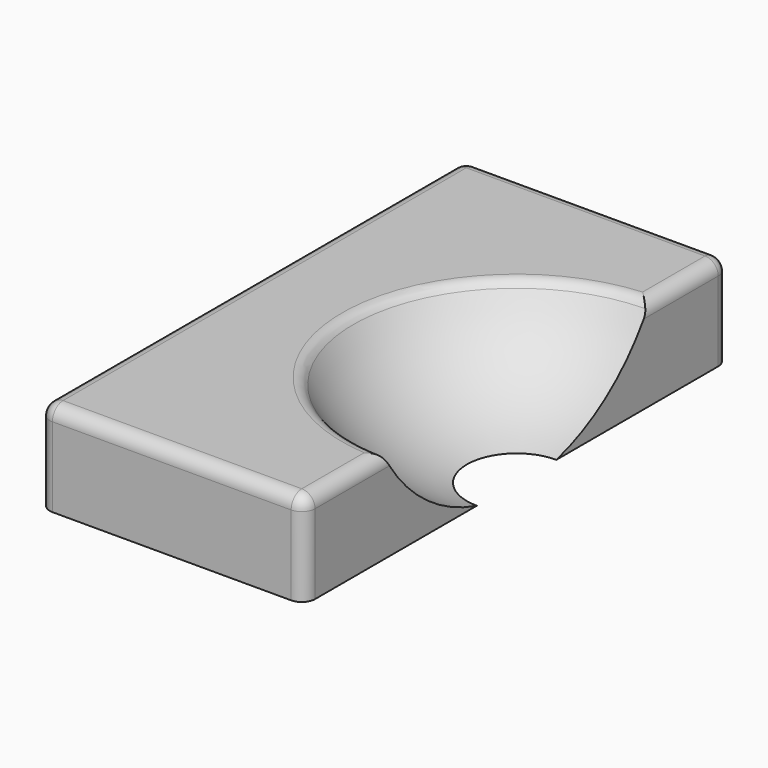
from build123d import *

# Parameters (mm, degrees)
F0_W         = 40
F0_H         = 80
F1_DEPTH     = 14
F4_T1_DEPTH  = 17.8405087492
F4_T3_DEPTH  = 17.8405087492
F4_T5_DEPTH  = 36
F4_T7_DEPTH  = 76
F4_T9_DEPTH  = 17
F4_S13_W     = 2
F4_S13_H     = 2
F4_T14_DEPTH = 2
F4_S19_W     = 2
F4_S19_H     = 2
F4_T20_DEPTH = 2
F4_S25_W     = 2
F4_S25_H     = 2
F4_T26_DEPTH = 2
F4_S31_W     = 2
F4_S31_H     = 2
F4_T32_DEPTH = 2
F4_T36_ANGLE = 193.2912055484


# Not quite as in the source:
# - a fillet or chamfer that OpenCascade refuses, or shapes differently, is made with other operations: its cross-section is extruded or revolved along the edge and cut away or added


with BuildPart() as f1:
    # F0 (on Top) → F1 (new body)
    with BuildSketch(Plane.XY):
        with Locations((20, -40)):
            Rectangle(F0_W, F0_H)
    extrude(amount=F1_DEPTH)

    # F2 (on face) → F3 (revolve, cut)
    with BuildSketch(Plane.YZ.offset(40)):
        with BuildLine():
            Line((-40, 0), (-32.5033340744, 0))
            ThreePointArc((-32.5033340744, 0), (-22.2346925053, 5.186748348), (-14.8405087492, 14))
            Line((-14.8405087492, 14), (-40, 14))
            Line((-40, 14), (-40, 0))
        make_face()
        with BuildLine():
            Line((-40, 14), (-14.8405087492, 14))
            ThreePointArc((-14.8405087492, 14), (-15.4345771459, 42.2458185159), (-40, 56.2))
            Line((-40, 56.2), (-40, 14))
        make_face()
        with BuildLine():
            Line((-40, 0), (-40, -1))
            ThreePointArc((-40, -1), (-36.2184659198, -0.7488976858), (-32.5033340744, 0))
            Line((-32.5033340744, 0), (-40, 0))
        make_face()
    revolve(axis=Axis((40, -40, 27.6), (0, 0, -1)), mode=Mode.SUBTRACT)

    # F4: fillet of radius 2 on 10 edges, made by hand

    # F4_s2 → F4_t1 (cut)
    with BuildSketch(Plane.XZ.offset(2)):
        with BuildLine():
            ThreePointArc((40, 12), (39.4142135624, 13.4142135624), (38, 14))
            Line((38, 14), (40, 14))
            Line((40, 14), (40, 12))
        make_face()
    extrude(amount=F4_T1_DEPTH, mode=Mode.SUBTRACT)

    # F4_s4 → F4_t3 (cut)
    with BuildSketch(Plane.XZ.offset(60.1594912508)):
        with BuildLine():
            ThreePointArc((38, 14), (39.4142135624, 13.4142135624), (40, 12))
            Line((40, 12), (40, 14))
            Line((40, 14), (38, 14))
        make_face()
    extrude(amount=F4_T3_DEPTH, mode=Mode.SUBTRACT)

    # F4_s6 → F4_t5 (cut)
    with BuildSketch(Plane.YZ.offset(2)):
        with BuildLine():
            ThreePointArc((-78, 14), (-79.4142135624, 13.4142135624), (-80, 12))
            Line((-80, 12), (-80, 14))
            Line((-80, 14), (-78, 14))
        make_face()
        with BuildLine():
            ThreePointArc((0, 12), (-0.5857864376, 13.4142135624), (-2, 14))
            Line((-2, 14), (0, 14))
            Line((0, 14), (0, 12))
        make_face()
    extrude(amount=F4_T5_DEPTH, mode=Mode.SUBTRACT)

    # F4_s8 → F4_t7 (cut)
    with BuildSketch(Plane.XZ.offset(2)):
        with BuildLine():
            ThreePointArc((0, 12), (0.5857864376, 13.4142135624), (2, 14))
            Line((2, 14), (0, 14))
            Line((0, 14), (0, 12))
        make_face()
    extrude(amount=F4_T7_DEPTH, mode=Mode.SUBTRACT)

    # F4_s10 → F4_t9 (cut)
    with BuildSketch(Plane.XY.offset(-5)):
        with BuildLine():
            ThreePointArc((38, -80), (39.4142135624, -79.4142135624), (40, -78))
            Line((40, -78), (40, -80))
            Line((40, -80), (38, -80))
        make_face()
        with BuildLine():
            ThreePointArc((0, -78), (0.5857864376, -79.4142135624), (2, -80))
            Line((2, -80), (0, -80))
            Line((0, -80), (0, -78))
        make_face()
        with BuildLine():
            ThreePointArc((38, 0), (39.4142135624, -0.5857864376), (40, -2))
            Line((40, -2), (40, 0))
            Line((40, 0), (38, 0))
        make_face()
        with BuildLine():
            ThreePointArc((2, 0), (0.5857864376, -0.5857864376), (0, -2))
            Line((0, -2), (0, 0))
            Line((0, 0), (2, 0))
        make_face()
    extrude(amount=F4_T9_DEPTH, mode=Mode.SUBTRACT)


with BuildPart() as f4_tool12:
    # F4_s13 → F4_t14 (new body)
    with BuildSketch(Plane.XZ.offset(2)):
        with Locations((39, 13)):
            Rectangle(F4_S13_W, F4_S13_H)
    extrude(amount=-F4_T14_DEPTH)

    # F4_s15 → F4_t16 (revolve, cut)
    with BuildSketch(Plane(origin=(38, -2, 12), x_dir=(-0.7071067812, 0, -0.7071067812), z_dir=(0.7071067812, 0, -0.7071067812))):
        with BuildLine():
            ThreePointArc((0, -2), (2, 0), (0, 2))
            Line((0, 2), (0, -2))
        make_face()
    revolve(axis=Axis((38, -2, 12), (0, 1, 0)), mode=Mode.SUBTRACT)


with BuildPart() as f1_1:
    add(f1.part)

    # F4_t11: cut F4_tool12
    add(f4_tool12.part, mode=Mode.SUBTRACT)


with BuildPart() as f4_tool18:
    # F4_s19 → F4_t20 (new body)
    with BuildSketch(Plane.XY.offset(12)):
        with Locations((39, -79)):
            Rectangle(F4_S19_W, F4_S19_H)
    extrude(amount=F4_T20_DEPTH)

    # F4_s21 → F4_t22 (revolve, cut)
    with BuildSketch(Plane(origin=(38, -78, 12), x_dir=(-0.7071067812, 0.7071067812, 0), z_dir=(0.7071067812, 0.7071067812, 0))):
        with BuildLine():
            ThreePointArc((0, -2), (2, 0), (0, 2))
            Line((0, 2), (0, -2))
        make_face()
    revolve(axis=Axis((38, -78, 12), (0, 0, 1)), mode=Mode.SUBTRACT)


with BuildPart() as f1_2:
    add(f1_1.part)

    # F4_t17: cut F4_tool18
    add(f4_tool18.part, mode=Mode.SUBTRACT)


with BuildPart() as f4_tool24:
    # F4_s25 → F4_t26 (new body)
    with BuildSketch(Plane.YZ.offset(2)):
        with Locations((-79, 13)):
            Rectangle(F4_S25_W, F4_S25_H)
    extrude(amount=-F4_T26_DEPTH)

    # F4_s27 → F4_t28 (revolve, cut)
    with BuildSketch(Plane(origin=(2, -78, 12), x_dir=(0, 0.7071067812, -0.7071067812), z_dir=(0, 0.7071067812, 0.7071067812))):
        with BuildLine():
            ThreePointArc((0, -2), (2, 0), (0, 2))
            Line((0, 2), (0, -2))
        make_face()
    revolve(axis=Axis((2, -78, 12), (-1, 0, 0)), mode=Mode.SUBTRACT)


with BuildPart() as f1_3:
    add(f1_2.part)

    # F4_t23: cut F4_tool24
    add(f4_tool24.part, mode=Mode.SUBTRACT)


with BuildPart() as f4_tool30:
    # F4_s31 → F4_t32 (new body)
    with BuildSketch(Plane.XZ.offset(2)):
        with Locations((1, 13)):
            Rectangle(F4_S31_W, F4_S31_H)
    extrude(amount=-F4_T32_DEPTH)

    # F4_s33 → F4_t34 (revolve, cut)
    with BuildSketch(Plane(origin=(2, -2, 12), x_dir=(0.7071067812, 0, -0.7071067812), z_dir=(0.7071067812, 0, 0.7071067812))):
        with BuildLine():
            ThreePointArc((0, -2), (2, 0), (0, 2))
            Line((0, 2), (0, -2))
        make_face()
    revolve(axis=Axis((2, -2, 12), (0, 1, 0)), mode=Mode.SUBTRACT)


with BuildPart() as f1_4:
    add(f1_3.part)

    # F4_t29: cut F4_tool30
    add(f4_tool30.part, mode=Mode.SUBTRACT)

    # F4_s35 → F4_t36 (revolve, cut)
    with BuildSketch(Plane(origin=(44.0622906263, -5.1337237407, 0), x_dir=(0, 0, 1), z_dir=(0.9932809704, -0.1157277578, 0))):
        with BuildLine():
            ThreePointArc((14, 8.7772353391), (13.7377018856, 9.7673828821), (13.0196078431, 10.4978165916))
            ThreePointArc((13.0196078431, 10.4978165916), (13.5070698024, 10.2153987353), (14, 9.9426372505))
            Line((14, 9.9426372505), (14, 8.7772353391))
        make_face()
    revolve(axis=Axis((40, -40, 14), (0, 0, 1)), revolution_arc=F4_T36_ANGLE, mode=Mode.SUBTRACT)


solid = f1_4.part
